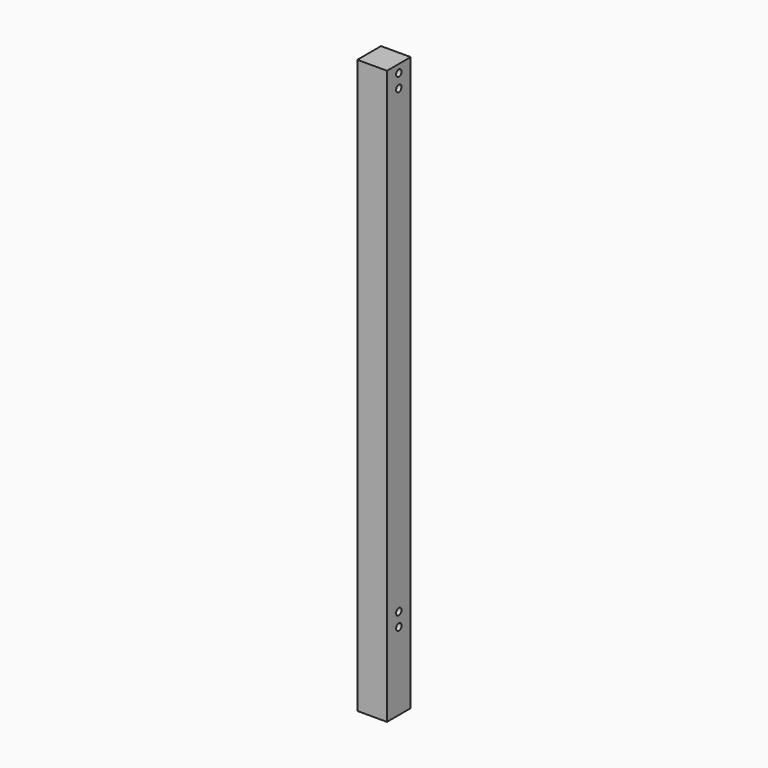
from build123d import *

# Parameters (mm, degrees)
F0_W     = 44
F0_H     = 44
F1_DEPTH = 850
F2_R     = 5
F3_DEPTH = 10
F4_R     = 5
F5_DEPTH = 10


# Not quite as in the source:
# - a feature names something its author has since deleted; it is built from what else it names


with BuildPart() as f1:
    # F0 (on Top) → F1 (new body)
    with BuildSketch(Plane.XY):
        with Locations((22, 22)):
            Rectangle(F0_W, F0_H)
    extrude(amount=F1_DEPTH)

    # F2 (on face) → F3 (cut)
    with BuildSketch(Plane(origin=(0, 44, 0), x_dir=(-1, 0, 0), z_dir=(0, 1, 0))):
        with Locations((-15, 115)):
            Circle(F2_R)
        with Locations((-15, 135)):
            Circle(F2_R)
        with Locations((-35, 435)):
            Circle(F2_R)
        with Locations((-15, 835)):
            Circle(F2_R)
        with Locations((-15, 815)):
            Circle(F2_R)
        with Locations((-35, 455)):
            Circle(F2_R)
    extrude(amount=-F3_DEPTH, mode=Mode.SUBTRACT)

    # F4 (on face) → F5 (cut)
    with BuildSketch(Plane.YZ.offset(44)):
        with Locations((22, 135)):
            Circle(F4_R)
        with Locations((22, 115)):
            Circle(F4_R)
        with Locations((22, 838)):
            Circle(F4_R)
        with Locations((22, 818)):
            Circle(F4_R)
    extrude(amount=-F5_DEPTH, mode=Mode.SUBTRACT)


solid = f1.part
